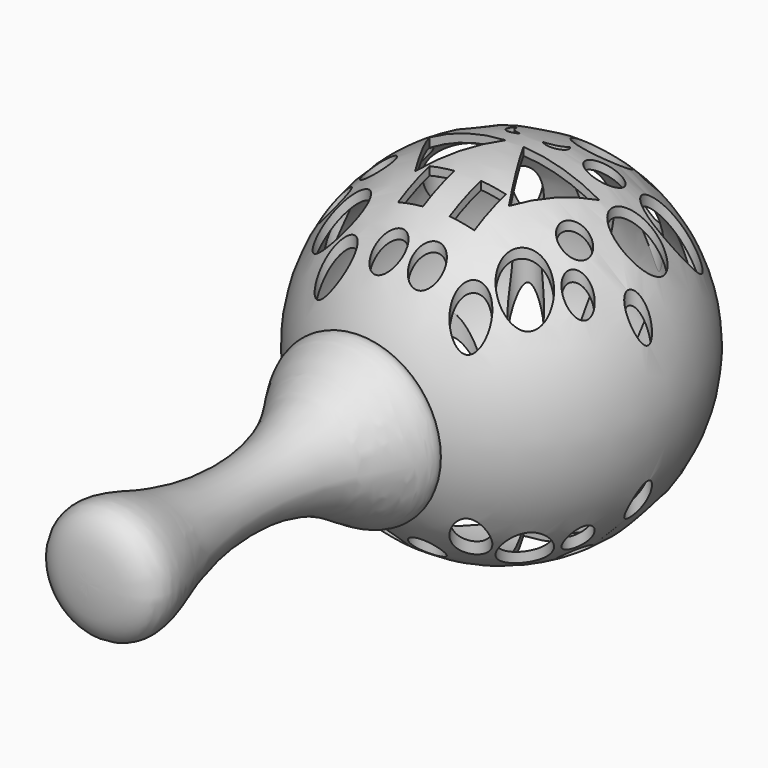
from build123d import *

# Parameters (mm, degrees)
F2_R     = 3.5726733295
F2_R_2   = 3.1476846975
F2_R_3   = 5.3134173971
F2_R_4   = 5.3134168119
F2_R_5   = 3.3196382076
F2_R_6   = 4.976917337
F2_R_7   = 3.6565833725
F2_R_8   = 5.1270092199
F2_R_9   = 2.8305898309
F2_W     = 5.4053803906
F2_H     = 8.5850171745
F2_R_10  = 3.155701501
F2_R_11  = 3.604365363
F2_R_12  = 1.5977453515
F2_R_13  = 2.3634321664
F3_DEPTH = 60


# Not quite as in the source:
# - the dataset's text gives a spline's control points without its knots; the knots are read off the source's solid


with BuildPart() as f1:
    # F0 (on Top) → F1 (revolve)
    with BuildSketch(Plane.XY):
        with BuildLine():
            add(Edge.make_bspline(
                [(9.9775328456, 1.3517104372), (13.7384674655, 0.8015647414), (22.6528101919, -0.4342342963), (4.8641593374, -18.4763260242), (6.3419887475, -53.8172578267), (17.9514139891, -75), (0, -75)],
                knots=[0, 0, 0, 0, 0.1623572539, 0.3967124596, 0.7431551679, 1, 1, 1, 1], degree=3))
            ThreePointArc((9.9775328456, 1.3517104372), (37.1605359125, 42.534339152), (0, 75))
            Line((0, 75), (0, 73.3))
            ThreePointArc((0, 73.3), (35.4759249511, 42.3061157771), (9.5252180232, 2.9904328974))
            Line((9.5252180232, 2.9904328974), (0, 2.9904328974))
            Line((0, 2.9904328974), (0, 0))
            Line((0, 0), (9.7314771098, -0.3303885815))
            add(Edge.make_bspline(
                [(9.7314771098, -0.3303885815), (10.4569375439, -0.4365081969), (11.8796087021, -0.6426364968), (13.4727354507, -0.9337030932), (14.5527718563, -1.205269162), (15.2401024887, -1.4276369114), (15.7765632301, -1.6607692795), (16.1337310372, -1.8820381572), (16.2709007745, -2.0167856567), (16.3097576615, -2.0717404519), (16.3189202628, -2.0910786035), (16.3209415162, -2.0958388647), (16.3317906209, -2.1435450189), (16.3356740738, -2.3373722403), (16.2374651856, -2.7874455763), (16.0070624339, -3.406044251), (15.6484939595, -4.1558980451), (15.0188640059, -5.2990568425), (13.9913533827, -6.9578879675), (12.5148578291, -9.2517480518), (10.9307066534, -11.8179323347), (9.6318529781, -14.1671336748), (8.6714058741, -16.1666688874), (7.788774332, -18.2449011378), (6.8617591886, -20.9425373579), (6.0122030218, -24.3227487862), (5.4161951008, -27.8214402001), (5.0624504972, -31.4171866769), (4.9004896107, -36.3120154265), (5.1835781488, -41.3149534056), (5.8757073901, -46.3406695738), (6.4717434549, -49.4734606826), (7.0423950815, -51.9638861834), (7.5165738258, -53.8214160027), (8.0347861056, -55.6647429192), (8.6003969094, -57.4957744264), (9.1889280186, -59.2797710037), (9.9541805879, -61.5816006678), (10.791817313, -64.2827010135), (11.2506757376, -66.6321952771), (11.2970221895, -68.1997605241), (11.1687904395, -69.1966102766), (10.8866256166, -70.018482038), (10.4428886146, -70.7200620696), (9.7640760506, -71.3730229222), (8.7409460517, -71.9912273951), (7.2960146522, -72.5357656205), (4.7529878426, -73.1040140177), (2.1148533623, -73.299999843), (0, -73.299999843)],
                knots=[0, 0, 0, 0, 0.03125, 0.0625, 0.078125, 0.09375, 0.109375, 0.125, 0.140625, 0.1484375, 0.15625, 0.1640625, 0.171875, 0.1875, 0.203125, 0.21875, 0.234375, 0.25, 0.28125, 0.3125, 0.34375, 0.375, 0.390625, 0.40625, 0.4375, 0.46875, 0.5, 0.53125, 0.5625, 0.625, 0.65625, 0.6875, 0.703125, 0.71875, 0.734375, 0.75, 0.765625, 0.78125, 0.8125, 0.84375, 0.859375, 0.875, 0.890625, 0.90625, 0.921875, 0.9375, 0.953125, 0.96875, 1, 1, 1, 1], degree=3))
            Line((0, -73.299999843), (0, -75))
        make_face()
    revolve(axis=Axis((0, 1.4952164487, 0), (0, -1, 0)))

    # F2 (on Top) → F3 (cut, symmetric)
    with BuildSketch(Plane.XY):
        with Locations((5.4470920004, 69.2130252719)):
            Circle(F2_R)
        with Locations((17.6886916161, 66.1923736334)):
            Circle(F2_R_2)
        with Locations((6.2420042232, 56.9714270532)):
            Circle(F2_R_3)
        with Locations((23.7300023437, 54.1097521782)):
            Circle(F2_R_4)
        with Locations((4.1752378456, 12.1385538951)):
            Circle(F2_R_5)
        with Locations((19.9144408107, 18.9747717232)):
            Circle(F2_R_6)
        with Locations((14.6680381149, 10.8666997403)):
            Circle(F2_R_7)
        with Locations((25.4788026214, 42.663063854)):
            Circle(F2_R_8)
        with Locations((26.4326930046, 25.3340452909)):
            Circle(F2_R_9)
        Polygon((18.4774885344, 41.073244065), (1.9556095433, 41.073244065), (10.2165490389, 26.7648771405), align=None)
        with Locations((5.6060738862, 24.0621902049)):
            Rectangle(F2_W, F2_H)
        with Locations((21.3452763855, 30.7394266129)):
            Circle(F2_R_10)
        with Locations((13.7141477317, 48.3864061534)):
            Circle(F2_R_11)
        with Locations((12.601274997, 61.8998594582)):
            Circle(F2_R_12)
        with Locations((32.632984221, 33.9190606028)):
            Circle(F2_R_13)
        with BuildLine():
            ThreePointArc((5.7650557719, 49.0223355591), (4.6025756051, 46.8461986258), (2.4264382664, 45.6837192178))
            ThreePointArc((2.4264382664, 45.6837192178), (5.6874584216, 45.761315431), (5.7650557719, 49.0223355591))
        make_face()
        with Locations((-5.4470920004, 69.2130252719)):
            Circle(F2_R)
        with Locations((-6.2420042232, 56.9714270532)):
            Circle(F2_R_3)
        with Locations((-12.601274997, 61.8998594582)):
            Circle(F2_R_12)
        with Locations((-17.6886916161, 66.1923736334)):
            Circle(F2_R_2)
        with Locations((-23.7300023437, 54.1097521782)):
            Circle(F2_R_4)
        with Locations((-13.7141477317, 48.3864061534)):
            Circle(F2_R_11)
        with BuildLine():
            ThreePointArc((-5.7650557719, 49.0223355591), (-5.6874584216, 45.761315431), (-2.4264382664, 45.6837192178))
            ThreePointArc((-2.4264382664, 45.6837192178), (-4.6025756051, 46.8461986258), (-5.7650557719, 49.0223355591))
        make_face()
        Polygon((-10.2165490389, 26.7648771405), (-1.9556095433, 41.073244065), (-18.4774885344, 41.073244065), align=None)
        with Locations((-25.4788026214, 42.663063854)):
            Circle(F2_R_8)
        with Locations((-32.632984221, 33.9190606028)):
            Circle(F2_R_13)
        with Locations((-21.3452763855, 30.7394266129)):
            Circle(F2_R_10)
        with Locations((-5.6060738862, 24.0621902049)):
            Rectangle(F2_W, F2_H)
        with Locations((-14.6680381149, 10.8666997403)):
            Circle(F2_R_7)
        with Locations((-4.1752378456, 12.1385538951)):
            Circle(F2_R_5)
        with Locations((-19.9144408107, 18.9747717232)):
            Circle(F2_R_6)
        with Locations((-26.4326930046, 25.3340452909)):
            Circle(F2_R_9)
    extrude(amount=F3_DEPTH, both=True, mode=Mode.SUBTRACT)


solid = f1.part
